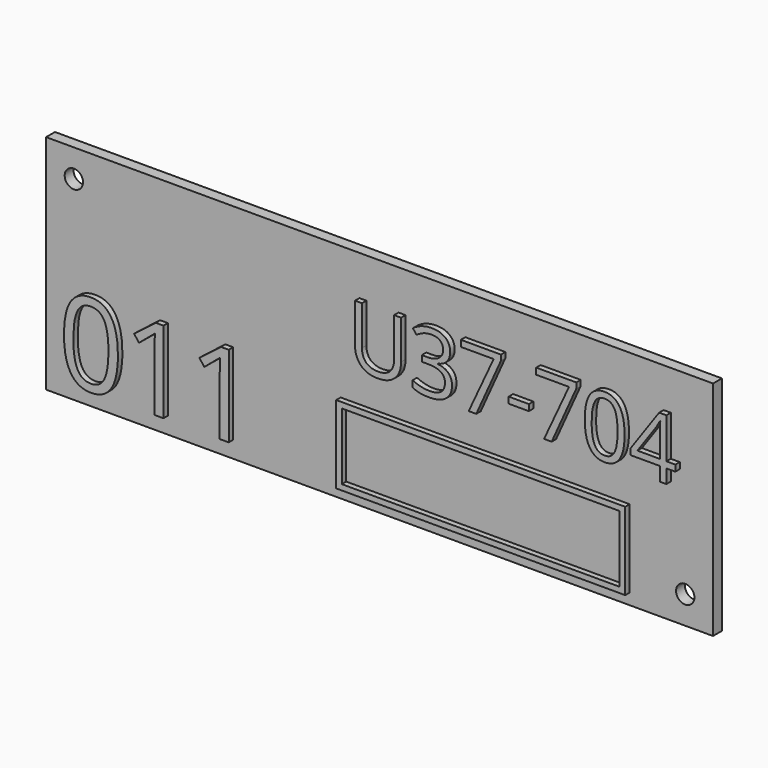
from build123d import *

# Parameters (mm, degrees)
F0_W         = 120
F0_H         = 40
F1_DEPTH     = 2
F3_D         = 3.3
F4_TEXT_SIZE = 15.1778656126
F5_DEPTH     = 1
F6_TEXT_SIZE = 20.5478077656
F7_DEPTH     = 1
F8_W         = 52
F8_H         = 14
F8_W_2       = 49.99999962
F8_H_2       = 11.99999962
F9_DEPTH     = 1


# Not quite as in the source:
# - Text() gives the source's letters only with a copy of the font that has no kerning and outlines rounded to 1/6400 em; it was checked with that copy


with BuildPart() as f1:
    # F0 (on Front) → F1 (new body)
    with BuildSketch(Plane.XZ):
        Rectangle(F0_W, F0_H)
    extrude(amount=F1_DEPTH)

    # F3 (through all)
    with Locations(Plane.XZ.offset(2)):
        with Locations((-55, 15), (55, -15)):
            Hole(F3_D / 2)

    # F4 (on face) → F5 (join)
    with BuildSketch(Plane.XZ.offset(2)):
        with Locations((-5, 2)):
            Text('U37-704', F4_TEXT_SIZE, font='Open Sans', text_align=(TextAlign.LEFT, TextAlign.BOTTOM))
    extrude(amount=F5_DEPTH)

    # F6 (on face) → F7 (join)
    with BuildSketch(Plane.XZ.offset(2)):
        with Locations((-57, -17)):
            Text('011', F6_TEXT_SIZE, font='Open Sans', text_align=(TextAlign.LEFT, TextAlign.BOTTOM))
    extrude(amount=F7_DEPTH)

    # F8 (on face) → F9 (join)
    with BuildSketch(Plane.XZ.offset(2)):
        with Locations((19, -11)):
            Rectangle(F8_W, F8_H)
        with Locations((19, -11)):
            Rectangle(F8_W_2, F8_H_2, mode=Mode.SUBTRACT)
    extrude(amount=F9_DEPTH)


solid = f1.part
